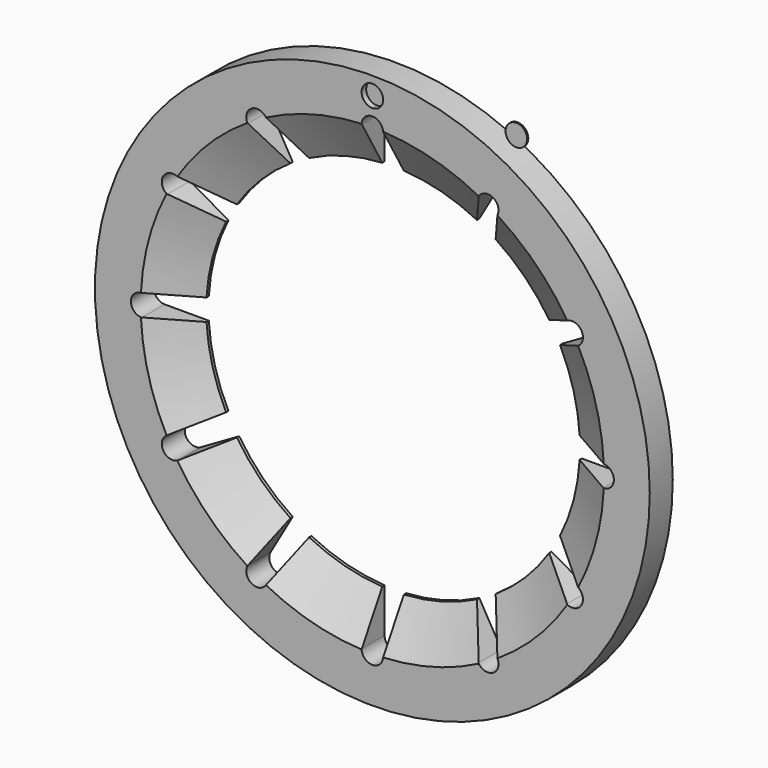
from build123d import *

# Parameters (mm, degrees)
F0_R        = 19.3
F1_DEPTH    = 2
F2_SIZE2    = 3.1176914536
F2_SIZE     = 1.8
F2_2_SIZE2  = 3.1176914536
F2_2_SIZE   = 1.8
F2_3_SIZE2  = 3.1176914536
F2_3_SIZE   = 1.8
F2_4_SIZE2  = 3.1176914536
F2_4_SIZE   = 1.8
F2_5_SIZE2  = 3.1176914536
F2_5_SIZE   = 1.8
F2_6_SIZE2  = 3.1176914536
F2_6_SIZE   = 1.8
F2_7_SIZE2  = 3.1176914536
F2_7_SIZE   = 1.8
F2_8_SIZE2  = 3.1176914536
F2_8_SIZE   = 1.8
F2_9_SIZE2  = 3.1176914536
F2_9_SIZE   = 1.8
F2_10_SIZE2 = 3.1176914536
F2_10_SIZE  = 1.8
F2_11_SIZE2 = 3.1176914536
F2_11_SIZE  = 1.8
F2_12_SIZE2 = 3.1176914536
F2_12_SIZE  = 1.8
F4_DEPTH    = 0.4
F3_R        = 0.75
F5_DEPTH    = 0.1


# Not quite as in the source:
# - a feature names something its author has since deleted; it is built from what else it names


with BuildPart() as f1:
    # F0 (on Front) → F1 (new body)
    with BuildSketch(Plane.XZ):
        Circle(F0_R)
        with BuildLine():
            ThreePointArc((-16.05, -0.75), (-16.8, 0), (-16.05, 0.75))
            Line((-16.05, 0.75), (-12.9783473524, 0.75))
            ThreePointArc((-12.9783473524, 0.75), (-12.5570357418, 3.3646475863), (-11.6145785063, 5.8396546234))
            Line((-11.6145785063, 5.8396546234), (-14.2747077307, 7.3754809472))
            ThreePointArc((-14.2747077307, 7.3754809472), (-14.5492267836, 8.4), (-13.5247077307, 8.6745190528))
            Line((-13.5247077307, 8.6745190528), (-10.8645785063, 7.138692729))
            ThreePointArc((-10.8645785063, 7.138692729), (-9.1923881554, 9.1923881554), (-7.138692729, 10.8645785063))
            Line((-7.138692729, 10.8645785063), (-8.6745190528, 13.5247077307))
            ThreePointArc((-8.6745190528, 13.5247077307), (-8.4, 14.5492267836), (-7.3754809472, 14.2747077307))
            Line((-7.3754809472, 14.2747077307), (-5.8396546234, 11.6145785063))
            ThreePointArc((-5.8396546234, 11.6145785063), (-3.3646475863, 12.5570357418), (-0.75, 12.9783473524))
            Line((-0.75, 12.9783473524), (-0.75, 16.05))
            ThreePointArc((-0.75, 16.05), (0, 16.8), (0.75, 16.05))
            Line((0.75, 16.05), (0.75, 12.9783473524))
            ThreePointArc((0.75, 12.9783473524), (3.3646475863, 12.5570357418), (5.8396546234, 11.6145785063))
            Line((5.8396546234, 11.6145785063), (7.3754809472, 14.2747077307))
            ThreePointArc((7.3754809472, 14.2747077307), (8.2191142838, 14.6241521005), (8.775, 13.8997077307))
            ThreePointArc((8.775, 13.8997077307), (8.7494443697, 13.7055934469), (8.6745190528, 13.5247077307))
            Line((8.6745190528, 13.5247077307), (7.138692729, 10.8645785063))
            ThreePointArc((7.138692729, 10.8645785063), (9.1923881554, 9.1923881554), (10.8645785063, 7.138692729))
            Line((10.8645785063, 7.138692729), (13.5247077307, 8.6745190528))
            ThreePointArc((13.5247077307, 8.6745190528), (14.2747077307, 8.6745190528), (14.6497077307, 8.025))
            ThreePointArc((14.6497077307, 8.025), (14.5492267836, 7.65), (14.2747077307, 7.3754809472))
            Line((14.2747077307, 7.3754809472), (11.6145785063, 5.8396546234))
            ThreePointArc((11.6145785063, 5.8396546234), (12.5570357418, 3.3646475863), (12.9783473524, 0.75))
            Line((12.9783473524, 0.75), (16.05, 0.75))
            ThreePointArc((16.05, 0.75), (16.5803300859, 0.5303300859), (16.8, 0))
            ThreePointArc((16.8, 0), (16.5803300859, -0.5303300859), (16.05, -0.75))
            Line((16.05, -0.75), (12.9783473524, -0.75))
            ThreePointArc((12.9783473524, -0.75), (12.5570357418, -3.3646475863), (11.6145785063, -5.8396546234))
            Line((11.6145785063, -5.8396546234), (14.2747077307, -7.3754809472))
            ThreePointArc((14.2747077307, -7.3754809472), (14.5492267836, -7.65), (14.6497077307, -8.025))
            ThreePointArc((14.6497077307, -8.025), (14.2747077307, -8.6745190528), (13.5247077307, -8.6745190528))
            Line((13.5247077307, -8.6745190528), (10.8645785063, -7.138692729))
            ThreePointArc((10.8645785063, -7.138692729), (9.1923881554, -9.1923881554), (7.138692729, -10.8645785063))
            Line((7.138692729, -10.8645785063), (8.6745190528, -13.5247077307))
            ThreePointArc((8.6745190528, -13.5247077307), (8.7494443697, -13.7055934469), (8.775, -13.8997077307))
            ThreePointArc((8.775, -13.8997077307), (8.2191142838, -14.6241521005), (7.3754809472, -14.2747077307))
            Line((7.3754809472, -14.2747077307), (5.8396546234, -11.6145785063))
            ThreePointArc((5.8396546234, -11.6145785063), (3.3646475863, -12.5570357418), (0.75, -12.9783473524))
            Line((0.75, -12.9783473524), (0.75, -16.05))
            ThreePointArc((0.75, -16.05), (0, -16.8), (-0.75, -16.05))
            Line((-0.75, -16.05), (-0.75, -12.9783473524))
            ThreePointArc((-0.75, -12.9783473524), (-3.3646475863, -12.5570357418), (-5.8396546234, -11.6145785063))
            Line((-5.8396546234, -11.6145785063), (-7.3754809472, -14.2747077307))
            ThreePointArc((-7.3754809472, -14.2747077307), (-8.4, -14.5492267836), (-8.6745190528, -13.5247077307))
            Line((-8.6745190528, -13.5247077307), (-7.138692729, -10.8645785063))
            ThreePointArc((-7.138692729, -10.8645785063), (-9.1923881554, -9.1923881554), (-10.8645785063, -7.138692729))
            Line((-10.8645785063, -7.138692729), (-13.5247077307, -8.6745190528))
            ThreePointArc((-13.5247077307, -8.6745190528), (-14.5492267836, -8.4), (-14.2747077307, -7.3754809472))
            Line((-14.2747077307, -7.3754809472), (-11.6145785063, -5.8396546234))
            ThreePointArc((-11.6145785063, -5.8396546234), (-12.5570357418, -3.3646475863), (-12.9783473524, -0.75))
            Line((-12.9783473524, -0.75), (-16.05, -0.75))
        make_face(mode=Mode.SUBTRACT)
    extrude(amount=F1_DEPTH)

    # F2
    f2_edges = [f1.edges().sort_by_distance(p)[0] for p in [
        (-9.192388, -2, 9.192388),
    ]]
    f2_side = f1.faces().sort_by_distance((-9.192388, -1, 9.192388))[0]
    chamfer(f2_edges, length=F2_SIZE, length2=F2_SIZE2, reference=f2_side)

    # F2#2
    f2_2_edges = [f1.edges().sort_by_distance(p)[0] for p in [
        (-3.364648, -2, 12.557036),
    ]]
    f2_2_side = f1.faces().sort_by_distance((-3.364648, -1, 12.557036))[0]
    chamfer(f2_2_edges, length=F2_2_SIZE, length2=F2_2_SIZE2, reference=f2_2_side)

    # F2#3
    f2_3_edges = [f1.edges().sort_by_distance(p)[0] for p in [
        (3.364648, -2, 12.557036),
    ]]
    f2_3_side = f1.faces().sort_by_distance((3.364648, -1, 12.557036))[0]
    chamfer(f2_3_edges, length=F2_3_SIZE, length2=F2_3_SIZE2, reference=f2_3_side)

    # F2#4
    f2_4_edges = [f1.edges().sort_by_distance(p)[0] for p in [
        (9.192388, -2, 9.192388),
    ]]
    f2_4_side = f1.faces().sort_by_distance((9.192388, -1, 9.192388))[0]
    chamfer(f2_4_edges, length=F2_4_SIZE, length2=F2_4_SIZE2, reference=f2_4_side)

    # F2#5
    f2_5_edges = [f1.edges().sort_by_distance(p)[0] for p in [
        (12.557036, -2, 3.364648),
    ]]
    f2_5_side = f1.faces().sort_by_distance((12.557036, -1, 3.364648))[0]
    chamfer(f2_5_edges, length=F2_5_SIZE, length2=F2_5_SIZE2, reference=f2_5_side)

    # F2#6
    f2_6_edges = [f1.edges().sort_by_distance(p)[0] for p in [
        (-12.557036, -2, 3.364648),
    ]]
    f2_6_side = f1.faces().sort_by_distance((-12.557036, -1, 3.364648))[0]
    chamfer(f2_6_edges, length=F2_6_SIZE, length2=F2_6_SIZE2, reference=f2_6_side)

    # F2#7
    f2_7_edges = [f1.edges().sort_by_distance(p)[0] for p in [
        (-12.557036, -2, -3.364648),
    ]]
    f2_7_side = f1.faces().sort_by_distance((-12.557036, -1, -3.364648))[0]
    chamfer(f2_7_edges, length=F2_7_SIZE, length2=F2_7_SIZE2, reference=f2_7_side)

    # F2#8
    f2_8_edges = [f1.edges().sort_by_distance(p)[0] for p in [
        (-9.192388, -2, -9.192388),
    ]]
    f2_8_side = f1.faces().sort_by_distance((-9.192388, -1, -9.192388))[0]
    chamfer(f2_8_edges, length=F2_8_SIZE, length2=F2_8_SIZE2, reference=f2_8_side)

    # F2#9
    f2_9_edges = [f1.edges().sort_by_distance(p)[0] for p in [
        (-3.364648, -2, -12.557036),
    ]]
    f2_9_side = f1.faces().sort_by_distance((-3.364648, -1, -12.557036))[0]
    chamfer(f2_9_edges, length=F2_9_SIZE, length2=F2_9_SIZE2, reference=f2_9_side)

    # F2#10
    f2_10_edges = [f1.edges().sort_by_distance(p)[0] for p in [
        (3.364648, -2, -12.557036),
    ]]
    f2_10_side = f1.faces().sort_by_distance((3.364648, -1, -12.557036))[0]
    chamfer(f2_10_edges, length=F2_10_SIZE, length2=F2_10_SIZE2, reference=f2_10_side)

    # F2#11
    f2_11_edges = [f1.edges().sort_by_distance(p)[0] for p in [
        (9.192388, -2, -9.192388),
    ]]
    f2_11_side = f1.faces().sort_by_distance((9.192388, -1, -9.192388))[0]
    chamfer(f2_11_edges, length=F2_11_SIZE, length2=F2_11_SIZE2, reference=f2_11_side)

    # F2#12
    f2_12_edges = [f1.edges().sort_by_distance(p)[0] for p in [
        (12.557036, -2, -3.364648),
    ]]
    f2_12_side = f1.faces().sort_by_distance((12.557036, -1, -3.364648))[0]
    chamfer(f2_12_edges, length=F2_12_SIZE, length2=F2_12_SIZE2, reference=f2_12_side)

    # F3 (on face) → F4 (cut)
    with BuildSketch(Plane.XZ.offset(2)):
        with BuildLine():
            ThreePointArc((0, 18.8), (-0.75, 18.05), (0, 17.3))
            Line((0, 17.3), (0, 18.8))
        make_face()
        with BuildLine():
            Line((0, 18.8), (0, 17.3))
            ThreePointArc((0, 17.3), (0.5303300859, 17.5196699141), (0.75, 18.05))
            ThreePointArc((0.75, 18.05), (0.5303300859, 18.5803300859), (0, 18.8))
        make_face()
    extrude(amount=-F4_DEPTH, mode=Mode.SUBTRACT)


with BuildPart() as f5:
    # F3 (on face) → F5 (new body)
    with BuildSketch(Plane.XZ.offset(2)):
        with Locations((10.0974785164, 18.974237144)):
            Circle(F3_R)
    extrude(amount=F5_DEPTH)


solid = Compound([f1.part, f5.part])
